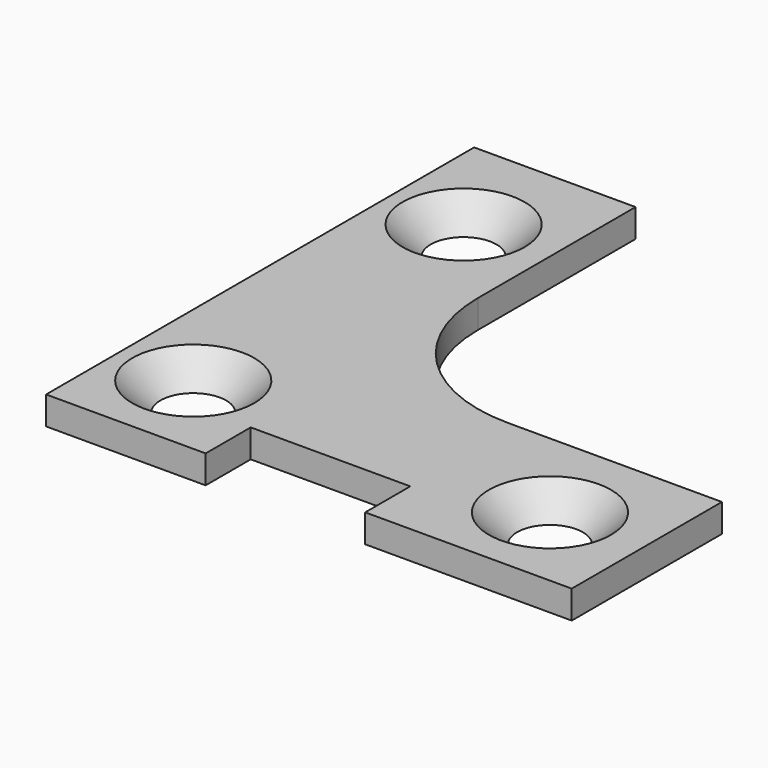
from build123d import *

# Parameters (mm, degrees)
F0_R     = 1.75
F1_DEPTH = 1.5
F2_SIZE  = 1.49999
F3_R     = 8


# Not quite as in the source:
# - a fillet or chamfer is up to 0.001 mm smaller than in the source, because OpenCascade refuses the exact size


with BuildPart() as f1:
    # F0 (on Top) → F1 (new body)
    with BuildSketch(Plane.XY):
        Polygon((0, 28.5), (0, 0), (8.5, 0), (8.5, 3), (17, 3), (17, 0), (28, 0), (28, 10), (8.6, 10), (8.6, 28.5), align=None)
        with Locations((4, 4.8)):
            Circle(F0_R, mode=Mode.SUBTRACT)
        with Locations((23, 4.8)):
            Circle(F0_R, mode=Mode.SUBTRACT)
        with Locations((4, 22.8)):
            Circle(F0_R, mode=Mode.SUBTRACT)
    extrude(amount=F1_DEPTH)

    # F2 (size 1.5 in the source; OpenCascade refuses exactly that, so slightly less here)
    f2_edges = [f1.edges().sort_by_distance(p)[0] for p in [
        (2.25, 22.8, 1.5),
        (2.25, 4.8, 1.5),
        (21.25, 4.8, 1.5),
    ]]
    chamfer(f2_edges, length=F2_SIZE)

    # F3
    f3_edges = [f1.edges().sort_by_distance(p)[0] for p in [
        (8.6, 10, 0.75),
    ]]
    fillet(f3_edges, radius=F3_R)


solid = f1.part
